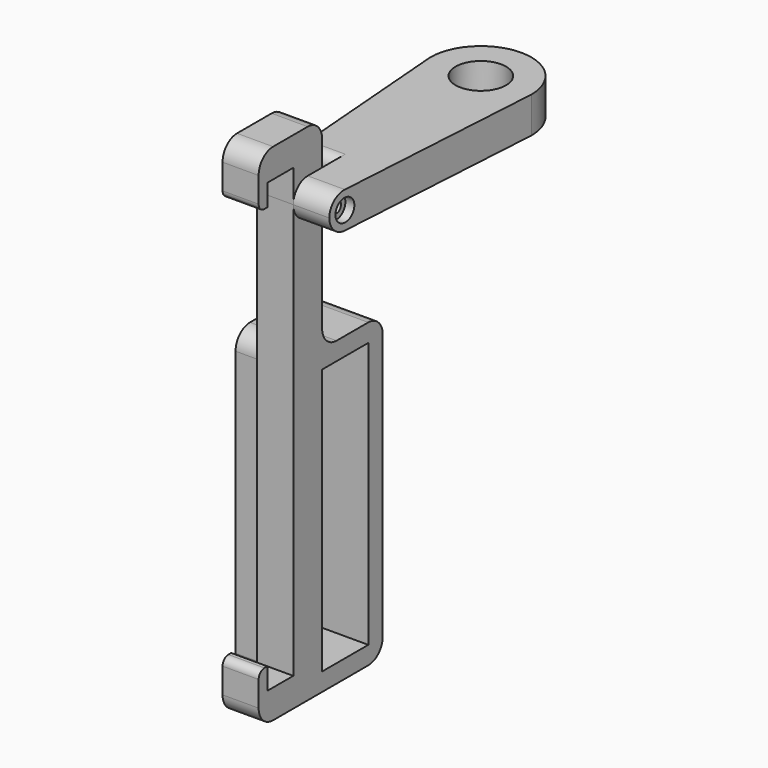
from build123d import *

# Parameters (mm, degrees)
F0_R      = 7
F1_DEPTH  = 10
F2_R      = 4.99999
F3_R      = 1.55
F4_DEPTH  = 11.4030769231
F5_START  = -8
F3_R_2    = 3.05
F5_DEPTH  = 4
F6_R      = 1.55
F7_DEPTH  = 10
F8_R      = 1.55
F9_DEPTH  = 2
F10_R     = 3
F11_W     = 16
F11_H     = 73.7
F12_DEPTH = 10


# Not quite as in the source:
# - a fillet or chamfer is up to 0.001 mm smaller than in the source, because OpenCascade refuses the exact size
# - ends of sketch curves that miss each other by under 0.0002 mm in the source are joined
# - a feature names something its author has since deleted; it is built from what else it names


with BuildPart() as f1:
    # F0 (on Top) → F1 (new body)
    with BuildSketch(Plane.XY):
        with BuildLine():
            Line((10, -65), (14, 0))
            ThreePointArc((14, 0), (0, 14), (-14, 0))
            Line((-14, 0), (-10, -50))
            Line((-10, -50), (0, -50))
            Line((0, -50), (0, -65))
            Line((0, -65), (10, -65))
        make_face()
        Circle(F0_R, mode=Mode.SUBTRACT)
    extrude(amount=F1_DEPTH)

    # F2 (radius 5 in the source; OpenCascade refuses exactly that, so slightly less here)
    f2_edges = [f1.edges().sort_by_distance(p)[0] for p in [
        (5, -65, 10),
        (5, -65, 0),
    ]]
    fillet(f2_edges, radius=F2_R)

    # F3 (on face) → F4 (cut, up to face)
    with BuildSketch(Plane(origin=(0, 0, 0), x_dir=(0, -1, 0), z_dir=(-1, 0, 0))):
        with Locations((60, 5)):
            Circle(F3_R)
    extrude(amount=-F4_DEPTH, mode=Mode.SUBTRACT)

    # F3 (on face) → F5 (cut)
    with BuildSketch(Plane(origin=(0, 0, 0), x_dir=(0, -1, 0), z_dir=(-1, 0, 0)).offset(F5_START)):
        with Locations((60, 5)):
            Circle(F3_R_2)
        with Locations((60, 5)):
            Circle(F3_R, mode=Mode.SUBTRACT)
    extrude(amount=-F5_DEPTH, mode=Mode.SUBTRACT)

    # F10
    f10_edges = [f1.edges().sort_by_distance(p)[0] for p in [
        (-5, -50, 10),
        (-5, -50, 0),
    ]]
    fillet(f10_edges, radius=F10_R)


with BuildPart() as f7:
    # F6 (on face) → F7 (new body)
    with BuildSketch(Plane(origin=(0, 0, 0), x_dir=(0, -1, 0), z_dir=(-1, 0, 0))):
        with BuildLine():
            ThreePointArc((60.00001, 0), (63.5355368349, 1.4644631651), (65, 4.99999))
            ThreePointArc((65, 4.99999), (63.5355368349, 8.5355368349), (60.00001, 10))
            Line((60.00001, 10), (55, 10))
            Line((55, 10), (55, 0))
            Line((55, 0), (60.00001, 0))
        make_face()
        with Locations((60, 5)):
            Circle(F6_R, mode=Mode.SUBTRACT)
        with BuildLine():
            Line((74, -110), (65, -110))
            Line((65, -110), (65, 5))
            ThreePointArc((65, 5), (63.5355368349, 1.4644631651), (60.00001, 0))
            Line((60.00001, 0), (55, 0))
            Line((55, 0), (55, -29.3))
            ThreePointArc((55, -29.3), (53.5355339059, -32.8355339059), (50, -34.3))
            Line((50, -34.3), (39, -34.3))
            ThreePointArc((39, -34.3), (35.4644660941, -35.7644660941), (34, -39.3))
            Line((34, -39.3), (34, -113))
            ThreePointArc((34, -113), (35.4644660941, -116.5355339059), (39, -118))
            Line((39, -118), (72, -118))
            ThreePointArc((72, -118), (75.5355339059, -116.5355339059), (77, -113))
            Line((77, -113), (77, -106))
            ThreePointArc((77, -106), (76.4142135624, -104.5857864376), (75, -104))
            Line((75, -104), (74, -104))
            Line((74, -104), (74, -110))
        make_face()
        Polygon((55, -39.3), (55, -110), (55, -113), (39, -113), (39, -39.3), align=None, mode=Mode.SUBTRACT)
        with BuildLine():
            ThreePointArc((60.00001, 10), (63.5355368349, 8.5355368349), (65, 5.00001))
            Line((65, 5.00001), (65, 14))
            Line((65, 14), (74, 14))
            Line((74, 14), (74, 8))
            Line((74, 8), (75, 8))
            ThreePointArc((75, 8), (76.4142135624, 8.5857864376), (77, 10))
            Line((77, 10), (77, 17))
            ThreePointArc((77, 17), (75.5355339059, 20.5355339059), (72, 22))
            Line((72, 22), (60, 22))
            ThreePointArc((60, 22), (56.4644660941, 20.5355339059), (55, 17))
            Line((55, 17), (55, 14))
            Line((55, 14), (55, 10))
            Line((55, 10), (60.00001, 10))
        make_face()
    extrude(amount=F7_DEPTH)

    # F8 (on face) → F9 (cut)
    with BuildSketch(Plane(origin=(-10, 0, 0), x_dir=(0, -1, 0), z_dir=(-1, 0, 0))):
        Polygon((62.8, 3.3834192463), (62.8, 6.6165807537), (60, 8.2331615075), (57.2, 6.6165807537), (57.2, 3.3834192463), (60, 1.7668384925), align=None)
        with Locations((60, 5)):
            Circle(F8_R, mode=Mode.SUBTRACT)
    extrude(amount=-F9_DEPTH, mode=Mode.SUBTRACT)

    # F11 (on face) → F12 (join)
    with BuildSketch(Plane(origin=(-10, 0, 0), x_dir=(0, -1, 0), z_dir=(-1, 0, 0))):
        with BuildLine():
            Line((34, -39.3), (34, -113))
            ThreePointArc((34, -113), (35.4644660941, -116.5355339059), (39, -118))
            Line((39, -118), (55, -118))
            ThreePointArc((55, -118), (58.5355339059, -116.5355339059), (60, -113))
            Line((60, -113), (60, -39.3))
            ThreePointArc((60, -39.3), (58.5355339059, -35.7644660941), (55, -34.3))
            Line((55, -34.3), (50, -34.3))
            Line((50, -34.3), (39, -34.3))
            ThreePointArc((39, -34.3), (35.4644660941, -35.7644660941), (34, -39.3))
        make_face()
        with Locations((47, -76.15)):
            Rectangle(F11_W, F11_H, mode=Mode.SUBTRACT)
    extrude(amount=F12_DEPTH)


solid = Compound([f1.part, f7.part])
